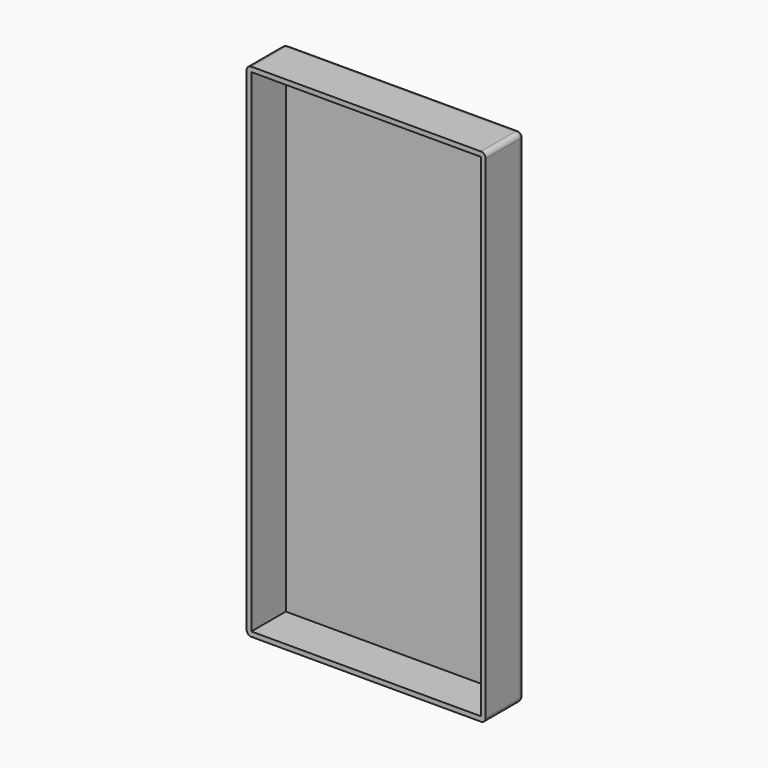
from build123d import *

# Parameters (mm, degrees)
F0_W     = 50
F0_H     = 105
F1_DEPTH = 10
F2_R     = 1
F3_R     = 1
F4_T     = 1


# Not quite as in the source:
# - a shell that OpenCascade refuses in one call is made with other operations: the cavity is built on its own and cut out


with BuildPart() as f1:
    # F0 (on Front) → F1 (new body)
    with BuildSketch(Plane.XZ):
        with Locations((-25, 52.5)):
            Rectangle(F0_W, F0_H)
    extrude(amount=F1_DEPTH)

    # F2
    f2_edges = [f1.edges().sort_by_distance(p)[0] for p in [
        (-50, -5, 105),
        (0, -5, 105),
        (0, -5, 0),
        (-50, -5, 0),
    ]]
    fillet(f2_edges, radius=F2_R)

    # F3
    f3_edges = [f1.edges().sort_by_distance(p)[0] for p in [
        (-25, 0, 105),
    ]]
    fillet(f3_edges, radius=F3_R)

    # F4: shell of thickness 1, made by hand


with BuildPart() as f4_core1:
    # F4_t2: copy of F1
    add(f1.part)

    # the walls: a layer under each face that stays
    f4_faces = [f4_core1.faces().sort_by_distance(p)[0] for p in [
        (0, -5.5, 52.5),
        (-25, -5.5, 0),
        (-25, 0, 52.5),
        (-25, -5.5, 105),
        (-50, -5.5, 52.5),
    ]]
    thicken(f4_faces, amount=-F4_T, mode=Mode.SUBTRACT)


with BuildPart() as f1_1:
    add(f1.part)

    # what is left inside the walls is the cavity
    f4_cavity = [f4_core1.part.solids().sort_by_distance(p)[0] for p in [
        (-25, -1.01, 35.333333),
    ]]
    add(f4_cavity, mode=Mode.SUBTRACT)


solid = f1_1.part
